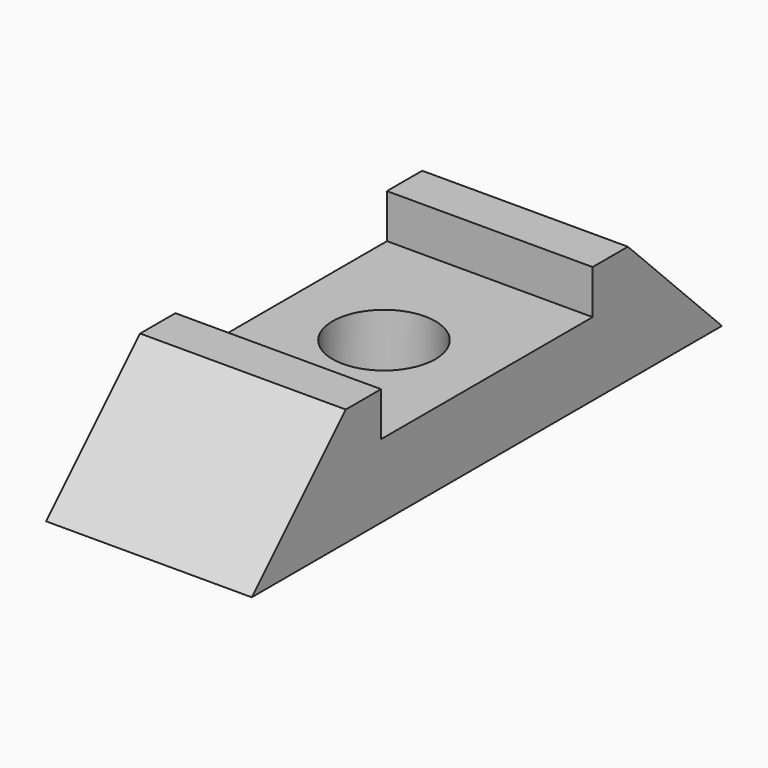
from build123d import *

# Parameters (mm, degrees)
F0_W     = 7
F0_H     = 20
F0_R     = 1.75
F1_DEPTH = 2.5
F2_W     = 7
F2_H     = 5.5
F3_DEPTH = 1.5
F4_SIZE  = 3.99999


# Not quite as in the source:
# - a fillet or chamfer is up to 0.001 mm smaller than in the source, because OpenCascade refuses the exact size


with BuildPart() as f1:
    # F0 (on Top) → F1 (new body)
    with BuildSketch(Plane.XY):
        Rectangle(F0_W, F0_H)
        Circle(F0_R, mode=Mode.SUBTRACT)
    extrude(amount=F1_DEPTH)

    # F2 (on face) → F3 (join)
    with BuildSketch(Plane.XY.offset(2.5)):
        with Locations((0, 7.25)):
            Rectangle(F2_W, F2_H)
        with Locations((0, -7.25)):
            Rectangle(F2_W, F2_H)
    extrude(amount=F3_DEPTH)

    # F4 (size 4 in the source; OpenCascade refuses exactly that, so slightly less here)
    f4_edges = [f1.edges().sort_by_distance(p)[0] for p in [
        (0, 10, 4),
        (0, -10, 4),
    ]]
    chamfer(f4_edges, length=F4_SIZE)


solid = f1.part
